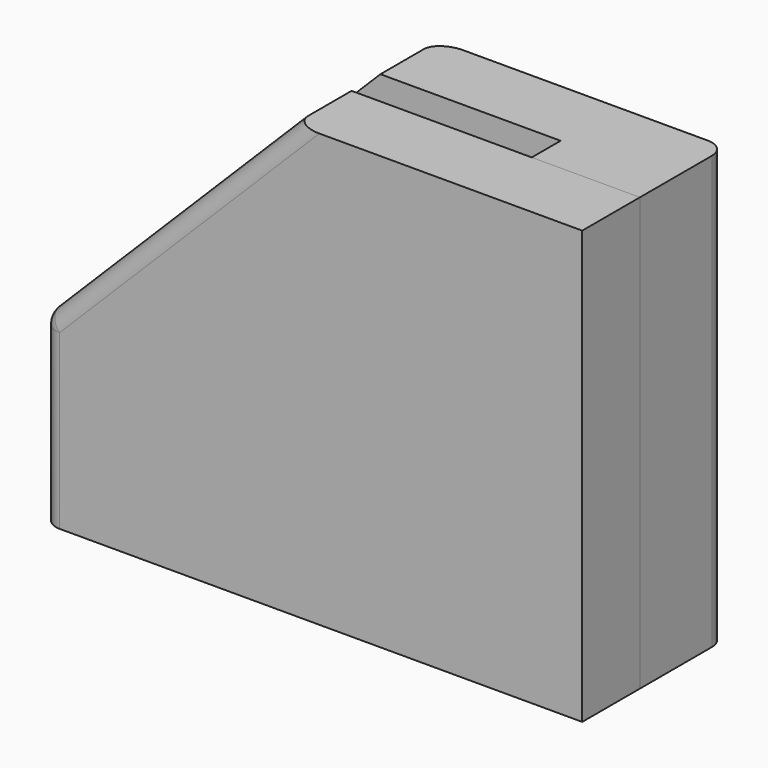
from build123d import *

# Parameters (mm, degrees)
F0_R     = 1.6054916764
F1_DEPTH = 3
F2_DEPTH = 1
F3_DEPTH = 0.5
F4_R     = 0.49999
F5_DEPTH = 2
F6_R     = 0.5
F7_R     = 0.5


# Not quite as in the source:
# - a fillet or chamfer is up to 0.001 mm smaller than in the source, because OpenCascade refuses the exact size


with BuildPart() as f1:
    # F0 (on Front) → F1 (new body)
    with BuildSketch(Plane.XZ):
        Polygon((0, 2), (0, 12), (-5, 12), (-12, 5), (-12, 2), align=None)
        with Locations((-4.2394283228, 5.5200844072)):
            Circle(F0_R, mode=Mode.SUBTRACT)
        with Locations((-4.2394283228, 5.5200844072)):
            Circle(F0_R)
        Polygon((3, 12), (0, 12), (0, 2), (-12, 2), (-12, 0), (0, 0), (3, 0), align=None)
    extrude(amount=-F1_DEPTH)

    # F0 (on Front) → F2 (cut)
    with BuildSketch(Plane.XZ):
        Polygon((0, 2), (0, 12), (-5, 12), (-12, 5), (-12, 2), align=None)
        with Locations((-4.2394283228, 5.5200844072)):
            Circle(F0_R, mode=Mode.SUBTRACT)
    extrude(amount=-F2_DEPTH, mode=Mode.SUBTRACT)

    # F0 (on Front) → F3 (cut)
    with BuildSketch(Plane.XZ):
        with Locations((-4.2394283228, 5.5200844072)):
            Circle(F0_R)
    extrude(amount=-F3_DEPTH, mode=Mode.SUBTRACT)

    # F4 (radius 0.5 in the source; OpenCascade refuses exactly that, so slightly less here)
    f4_edges = [f1.edges().sort_by_distance(p)[0] for p in [
        (-5.84492, 0.5, 5.520084),
    ]]
    fillet(f4_edges, radius=F4_R)

    # F7
    f7_edges = [f1.edges().sort_by_distance(p)[0] for p in [
        (-8.5, 3, 8.5),
        (-12, 2, 5),
        (-12, 3, 2.5),
        (3, 3, 6),
    ]]
    fillet(f7_edges, radius=F7_R)


with BuildPart() as f5:
    # F0 (on Front) → F5 (new body)
    with BuildSketch(Plane.XZ):
        Polygon((0, 2), (0, 12), (-5, 12), (-12, 5), (-12, 2), align=None)
        with Locations((-4.2394283228, 5.5200844072)):
            Circle(F0_R, mode=Mode.SUBTRACT)
        Polygon((3, 12), (0, 12), (0, 2), (-12, 2), (-12, 0), (0, 0), (3, 0), align=None)
        with Locations((-4.2394283228, 5.5200844072)):
            Circle(F0_R)
    extrude(amount=F5_DEPTH)

    # F6
    f6_edges = [f5.edges().sort_by_distance(p)[0] for p in [
        (-8.5, -2, 8.5),
        (-12, -2, 2.5),
        (-12, -1, 5),
    ]]
    fillet(f6_edges, radius=F6_R)


solid = Compound([f1.part, f5.part])
